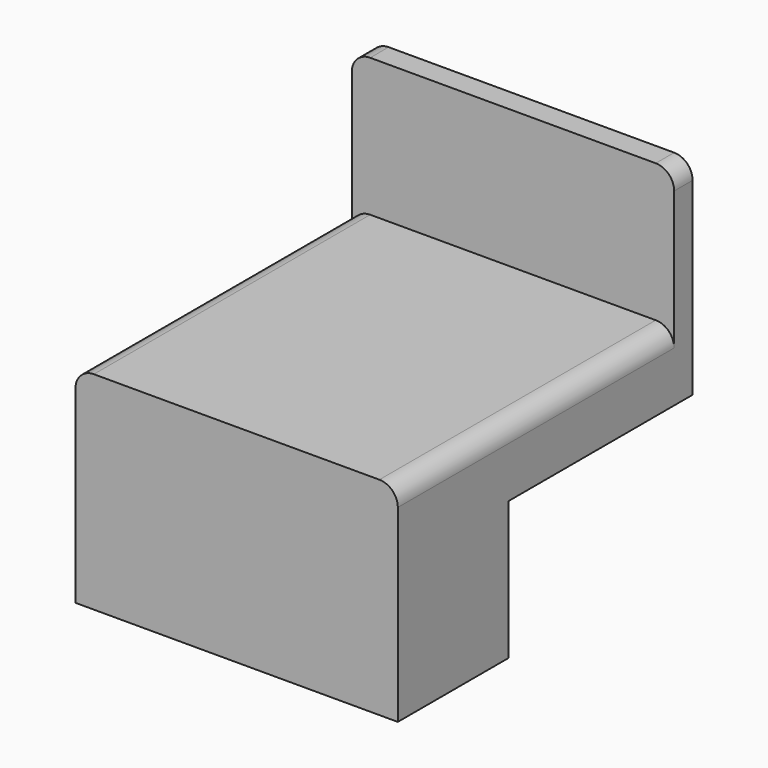
from build123d import *

# Parameters (mm, degrees)
F1_DEPTH = 38.1
F2_W     = 88.9
F2_H     = 101.6
F3_DEPTH = 19.05
F4_W     = 88.9
F4_H     = 6.35
F5_DEPTH = 38.1
F6_R     = 5.08


# Not quite as in the source:
# - a feature names something its author has since deleted; it is built from what else it names


with BuildPart() as f1:
    # F0 (on Top) → F1 (new body)
    with BuildSketch(Plane.XY):
        Polygon((-31.983944577, 23.2039450469), (-31.983944577, -40.2960549531), (56.916055423, -40.2960549531), (56.916055423, -2.1960549531), align=None)
    extrude(amount=F1_DEPTH)

    # F2 (on face) → F3 (join)
    with BuildSketch(Plane.XY.offset(38.1)):
        with Locations((12.466055423, 10.5039450469)):
            Rectangle(F2_W, F2_H)
    extrude(amount=F3_DEPTH)

    # F4 (on face) → F5 (join)
    with BuildSketch(Plane.XY.offset(57.15)):
        with Locations((12.466055423, 58.1289450469)):
            Rectangle(F4_W, F4_H)
    extrude(amount=F5_DEPTH)

    # F6
    f6_edges = [f1.edges().sort_by_distance(p)[0] for p in [
        (56.916055, 7.328945, 57.15),
        (-31.983945, 7.328945, 57.15),
        (-31.983945, 58.128945, 95.25),
        (56.916055, 58.128945, 95.25),
    ]]
    fillet(f6_edges, radius=F6_R)


solid = f1.part
